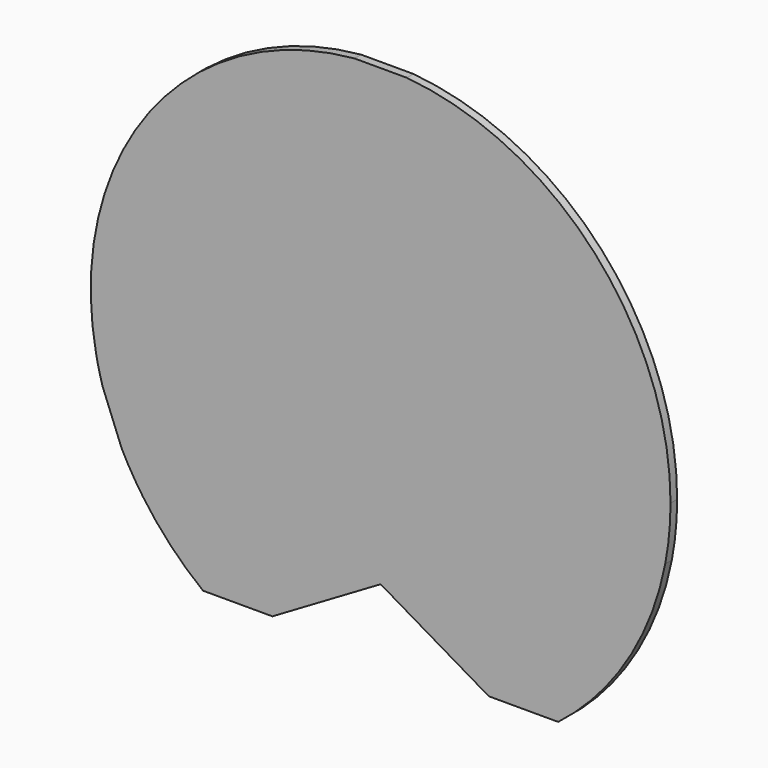
from build123d import *

# Parameters (mm, degrees)
F0_W     = 40
F0_H     = 40
F0_W_2   = 9.4724982
F0_H_2   = 96
F0_W_3   = 9.4725108908
F1_DEPTH = 3


# Not quite as in the source:
# - ends of sketch curves that miss each other by under 0.0002 mm in the source are joined


with BuildPart() as f1:
    # F0 (on Front) → F1 (new body)
    with BuildSketch(Plane.XZ):
        with BuildLine():
            ThreePointArc((86.0931563339, 18.3499035886), (87.5338209496, 28.3038164709), (88.0155156934, 38.3499035886))
            ThreePointArc((88.0155156934, 38.3499035886), (60.5384552721, 109.1679368787), (-7.5119860033, 142.9217534139))
            Line((-7.5119860033, 142.9217534139), (-7.5119861066, 46.9217522737))
            Line((-7.5119861066, 46.9217522737), (-16.9844843066, 46.9217522737))
            Line((-16.9844843066, 46.9217522737), (-16.9844843066, 38.3499035886))
            Line((-16.9844843066, 38.3499035886), (-16.9844843066, 18.3499035886))
            Line((-16.9844843066, 18.3499035886), (7.9387861441, 18.3499035886))
            Line((7.9387861441, 18.3499035886), (-12.4932068051, 26.3993963716))
            Line((-12.4932068051, 26.3993963716), (-8.6108822672, 35.0509963625))
            Line((-8.6108822672, 35.0509963625), (-5.9856059721, 42.9176116083))
            Line((-5.9856059721, 42.9176116083), (56.3745017477, 18.3499035886))
            Line((56.3745017477, 18.3499035886), (86.0931563339, 18.3499035886))
        make_face()
        with Locations((38.3114193761, 61.7765981326)):
            Rectangle(F0_W, F0_H, mode=Mode.SUBTRACT)
        with Locations((-12.2482352066, 94.9217522737)):
            Rectangle(F0_W_2, F0_H_2)
        with BuildLine():
            ThreePointArc((69.1839553915, -21.6500964114), (79.7291121051, -2.533837301), (86.0931563339, 18.3499035886))
            Line((86.0931563339, 18.3499035886), (56.3745017477, 18.3499035886))
            Line((56.3745017477, 18.3499035886), (83.3328157811, 7.7292678634))
            Line((83.3328157811, 7.7292678634), (80.2973141438, 0.0242670983))
            Line((80.2973141438, 0.0242670983), (76.8252149481, -8.7889473734))
            Line((76.8252149481, -8.7889473734), (7.9387861441, 18.3499035886))
            Line((7.9387861441, 18.3499035886), (-16.9844843066, 18.3499035886))
            Line((-16.9844843066, 18.3499035886), (69.1839553915, -21.6500964114))
        make_face()
        with Locations((-21.720739752, 94.9217522737)):
            Rectangle(F0_W_3, F0_H_2)
        with BuildLine():
            ThreePointArc((47.3344412398, -44.6445288546), (59.1325161296, -33.9771469845), (69.1839553915, -21.6500964114))
            Line((69.1839553915, -21.6500964114), (-16.9844843066, 18.3499035886))
            Line((-16.9844843066, 18.3499035886), (-103.1529240046, -21.6500964114))
            ThreePointArc((-103.1529240046, -21.6500964114), (-93.1014847427, -33.9771469845), (-81.3034098529, -44.6445288546))
            Line((-81.3034098529, -44.6445288546), (-56.1818756669, -44.6445288546))
            Line((-56.1818756669, -44.6445288546), (-16.9844843066, -21.6500964114))
            Line((-16.9844843066, -21.6500964114), (22.2130476509, -44.6445288546))
            Line((22.2130476509, -44.6445288546), (47.3344412398, -44.6445288546))
        make_face()
        Polygon((83.3328157811, 7.7292678634), (56.3745017477, 18.3499035886), (7.9387861441, 18.3499035886), (76.8252149481, -8.7889473734), (80.2973141438, 0.0242670983), align=None)
        Polygon((7.9387861441, 18.3499035886), (56.3745017477, 18.3499035886), (-5.9856059721, 42.9176116083), (-8.6108822672, 35.0509963625), (-12.4932068051, 26.3993963716), align=None)
        with BuildLine():
            Line((-26.4569951974, 46.9217522737), (-26.4569951974, 142.9217522737))
            ThreePointArc((-26.4569951974, 142.9217522737), (-100.9274442474, 101.4258853595), (-120.062124947, 18.3499035886))
            Line((-120.062124947, 18.3499035886), (-93.5930420098, 18.3499035886))
            Line((-93.5930420098, 18.3499035886), (-28.4441302912, 44.0163031416))
            Line((-28.4441302912, 44.0163031416), (-25.3580863459, 35.0509963625))
            Line((-25.3580863459, 35.0509963625), (-21.5126400611, 26.4221312691))
            Line((-21.5126400611, 26.4221312691), (-42.002340903, 18.3499035886))
            Line((-42.002340903, 18.3499035886), (-16.9844843066, 18.3499035886))
            Line((-16.9844843066, 18.3499035886), (-16.9844843066, 38.3499035886))
            Line((-16.9844843066, 38.3499035886), (-16.9844843066, 46.9217522737))
            Line((-16.9844843066, 46.9217522737), (-26.4569951974, 46.9217522737))
        make_face()
        with Locations((-72.2803842399, 61.7765981326)):
            Rectangle(F0_W, F0_H, mode=Mode.SUBTRACT)
        with BuildLine():
            Line((-103.1529240046, -21.6500964114), (-16.9844843066, 18.3499035886))
            Line((-16.9844843066, 18.3499035886), (-42.002340903, 18.3499035886))
            Line((-42.002340903, 18.3499035886), (-110.8216826256, -8.7625174025))
            ThreePointArc((-110.8216826256, -8.7625174025), (-107.2176813721, -15.3433934543), (-103.1529240046, -21.6500964114))
        make_face()
        with BuildLine():
            Line((-93.5930420098, 18.3499035886), (-120.062124947, 18.3499035886))
            ThreePointArc((-120.062124947, 18.3499035886), (-119.0172144252, 13.5643839342), (-117.750256284, 8.8328034975))
            Line((-117.750256284, 8.8328034975), (-93.5930420098, 18.3499035886))
        make_face()
        with BuildLine():
            Line((-110.8216826256, -8.7625174025), (-42.002340903, 18.3499035886))
            Line((-42.002340903, 18.3499035886), (-93.5930420098, 18.3499035886))
            Line((-93.5930420098, 18.3499035886), (-117.750256284, 8.8328034975))
            ThreePointArc((-117.750256284, 8.8328034975), (-117.7294799239, 8.7619692561), (-117.7086537702, 8.6911496387))
            Line((-117.7086537702, 8.6911496387), (-114.2904528488, 0.0147449249))
            Line((-114.2904528488, 0.0147449249), (-110.8722519274, -8.6616597888))
            ThreePointArc((-110.8722519274, -8.6616597888), (-110.8469808232, -8.7120953879), (-110.8216826256, -8.7625174025))
        make_face()
        Polygon((-93.5930420098, 18.3499035886), (-42.002340903, 18.3499035886), (-21.5126400611, 26.4221312691), (-25.3580863459, 35.0509963625), (-28.4441302912, 44.0163031416), align=None)
        with Locations((38.3114193761, 61.7765981326)):
            Rectangle(F0_W, F0_H)
        with Locations((-72.2803842399, 61.7765981326)):
            Rectangle(F0_W, F0_H)
    extrude(amount=F1_DEPTH)


solid = f1.part
